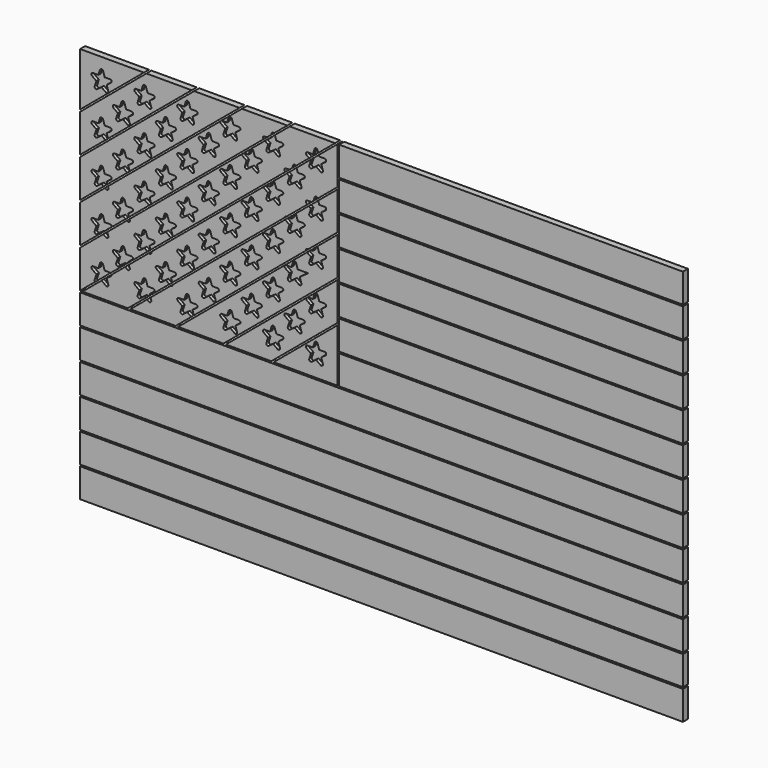
from build123d import *

# Parameters (mm, degrees)
F0_W     = 1219.2
F0_H     = 58.7375
F3_DEPTH = 12.7
F0_W_2   = 695.325
F4_START = 6.35
F4_DEPTH = 8.89
F5_R     = 3.175
F5_2_R   = 3.175
F5_3_R   = 3.175
F5_4_R   = 3.175
F5_5_R   = 3.175
F5_6_R   = 3.175
F5_7_R   = 3.175
F5_8_R   = 3.175
F5_9_R   = 3.175
F5_10_R  = 3.175
F5_11_R  = 3.175
F5_12_R  = 3.175
F5_13_R  = 3.175
F5_14_R  = 3.175
F5_15_R  = 3.175
F5_16_R  = 3.175
F5_17_R  = 3.175
F5_18_R  = 3.175
F5_19_R  = 3.175
F5_20_R  = 3.175
F5_21_R  = 3.175
F5_22_R  = 3.175
F5_23_R  = 3.175
F5_24_R  = 3.175
F5_25_R  = 3.175
F5_26_R  = 3.175
F5_27_R  = 3.175
F5_28_R  = 3.175
F5_29_R  = 3.175
F5_30_R  = 3.175
F5_31_R  = 3.175
F5_32_R  = 3.175
F5_33_R  = 3.175
F5_34_R  = 3.175
F5_35_R  = 3.175
F5_36_R  = 3.175
F5_37_R  = 3.175
F5_38_R  = 3.175
F5_39_R  = 3.175
F5_40_R  = 3.175
F5_41_R  = 3.175
F5_42_R  = 3.175
F5_43_R  = 3.175
F5_44_R  = 3.175
F5_45_R  = 3.175
F5_46_R  = 3.175
F5_47_R  = 3.175
F5_48_R  = 3.175
F5_49_R  = 3.175
F5_50_R  = 3.175


# Not quite as in the source:
# - a feature names something its author has since deleted; it is built from what else it names


with BuildPart() as f3:
    # F0 (on Front) → F3 (new body)
    with BuildSketch(Plane.XZ):
        with Locations((609.6, 277.01875)):
            Rectangle(F0_W, F0_H)
    extrude(amount=F3_DEPTH)


with BuildPart() as f3b:
    # F0 (on Front) → F3, piece 2 (new body)
    with BuildSketch(Plane.XZ):
        with Locations((609.6, 215.10625)):
            Rectangle(F0_W, F0_H)
    extrude(amount=F3_DEPTH)


with BuildPart() as f3c:
    # F0 (on Front) → F3, piece 3 (new body)
    with BuildSketch(Plane.XZ):
        with Locations((609.6, 153.19375)):
            Rectangle(F0_W, F0_H)
    extrude(amount=F3_DEPTH)


with BuildPart() as f3d:
    # F0 (on Front) → F3, piece 4 (new body)
    with BuildSketch(Plane.XZ):
        with Locations((609.6, 91.28125)):
            Rectangle(F0_W, F0_H)
    extrude(amount=F3_DEPTH)


with BuildPart() as f3e:
    # F0 (on Front) → F3, piece 5 (new body)
    with BuildSketch(Plane.XZ):
        with Locations((609.6, 29.36875)):
            Rectangle(F0_W, F0_H)
    extrude(amount=F3_DEPTH)


with BuildPart() as f3f:
    # F0 (on Front) → F3, piece 6 (new body)
    with BuildSketch(Plane.XZ):
        with Locations((609.6, 338.93125)):
            Rectangle(F0_W, F0_H)
    extrude(amount=F3_DEPTH)


with BuildPart() as f3g:
    # F0 (on Front) → F3, piece 7 (new body)
    with BuildSketch(Plane.XZ):
        with Locations((871.5375, 400.84375)):
            Rectangle(F0_W_2, F0_H)
    extrude(amount=F3_DEPTH)


with BuildPart() as f3h:
    # F0 (on Front) → F3, piece 8 (new body)
    with BuildSketch(Plane.XZ):
        with Locations((871.5375, 462.75625)):
            Rectangle(F0_W_2, F0_H)
    extrude(amount=F3_DEPTH)


with BuildPart() as f3i:
    # F0 (on Front) → F3, piece 9 (new body)
    with BuildSketch(Plane.XZ):
        with Locations((871.5375, 524.66875)):
            Rectangle(F0_W_2, F0_H)
    extrude(amount=F3_DEPTH)


with BuildPart() as f3j:
    # F0 (on Front) → F3, piece 10 (new body)
    with BuildSketch(Plane.XZ):
        with Locations((871.5375, 586.58125)):
            Rectangle(F0_W_2, F0_H)
    extrude(amount=F3_DEPTH)


with BuildPart() as f3k:
    # F0 (on Front) → F3, piece 11 (new body)
    with BuildSketch(Plane.XZ):
        with Locations((871.5375, 648.49375)):
            Rectangle(F0_W_2, F0_H)
    extrude(amount=F3_DEPTH)


with BuildPart() as f3l:
    # F0 (on Front) → F3, piece 12 (new body)
    with BuildSketch(Plane.XZ):
        with Locations((871.5375, 710.40625)):
            Rectangle(F0_W_2, F0_H)
    extrude(amount=F3_DEPTH)


with BuildPart() as f3m:
    # F0 (on Front) → F3, piece 13 (new body)
    with BuildSketch(Plane.XZ):
        with Locations((871.5375, 772.31875)):
            Rectangle(F0_W_2, F0_H)
    extrude(amount=F3_DEPTH)


with BuildPart() as f3n:
    # F0 (on Front) → F3, piece 14 (new body)
    with BuildSketch(Plane.XZ):
        Polygon((520.7, 371.475), (520.7, 479.188347446), (391.5720757397, 371.475), align=None)
    extrude(amount=F3_DEPTH)


with BuildPart() as f3o:
    # F0 (on Front) → F3, piece 15 (new body)
    with BuildSketch(Plane.XZ):
        Polygon((386.6154671861, 371.475), (520.7, 483.3229519659), (520.7, 559.8131355845), (294.9182089432, 371.475), align=None)
    extrude(amount=F3_DEPTH)


with BuildPart() as f3p:
    # F0 (on Front) → F3, piece 16 (new body)
    with BuildSketch(Plane.XZ):
        Polygon((520.7, 563.9477401044), (520.7, 640.437923723), (198.2643421467, 371.475), (289.9616003895, 371.475), align=None)
    extrude(amount=F3_DEPTH)


with BuildPart() as f3q:
    # F0 (on Front) → F3, piece 17 (new body)
    with BuildSketch(Plane.XZ):
        Polygon((520.7, 644.5725282429), (520.7, 721.0627118615), (101.6104753502, 371.475), (193.307733593, 371.475), align=None)
    extrude(amount=F3_DEPTH)


with BuildPart() as f3r:
    # F0 (on Front) → F3, piece 18 (new body)
    with BuildSketch(Plane.XZ):
        Polygon((520.7, 725.1973163814), (520.7, 801.6875), (4.9566085537, 371.475), (96.6538667965, 371.475), align=None)
    extrude(amount=F3_DEPTH)


with BuildPart() as f3s:
    # F0 (on Front) → F3, piece 19 (new body)
    with BuildSketch(Plane.XZ):
        Polygon((0, 371.475), (515.7433914463, 801.6875), (424.0461332035, 801.6875), (0, 447.9651836186), align=None)
    extrude(amount=F3_DEPTH)


with BuildPart() as f3t:
    # F0 (on Front) → F3, piece 20 (new body)
    with BuildSketch(Plane.XZ):
        Polygon((0, 528.5899717571), (0, 452.0997881385), (419.0895246498, 801.6875), (327.392266407, 801.6875), align=None)
    extrude(amount=F3_DEPTH)


with BuildPart() as f3u:
    # F0 (on Front) → F3, piece 21 (new body)
    with BuildSketch(Plane.XZ):
        Polygon((0, 532.724576277), (322.4356578533, 801.6875), (230.7383996105, 801.6875), (0, 609.2147598956), align=None)
    extrude(amount=F3_DEPTH)


with BuildPart() as f3v:
    # F0 (on Front) → F3, piece 22 (new body)
    with BuildSketch(Plane.XZ):
        Polygon((0, 613.3493644155), (225.7817910568, 801.6875), (134.0845328139, 801.6875), (0, 689.8395480341), align=None)
    extrude(amount=F3_DEPTH)


with BuildPart() as f3w:
    # F0 (on Front) → F3, piece 23 (new body)
    with BuildSketch(Plane.XZ):
        Polygon((0, 693.974152554), (129.1279242603, 801.6875), (0, 801.6875), align=None)
    extrude(amount=F3_DEPTH)


with BuildPart() as f4:
    # F2 (on Front) → F4 (new body)
    with BuildSketch(Plane.XZ.offset(F4_START)):
        Polygon((69.9856764157, 606.4772193857), (86.78164, 618.6802012285), (103.5776035843, 606.4772193857), (97.1621163689, 626.2220587715), (113.9580799531, 638.4250406143), (93.1971272154, 638.4250406143), (86.78164, 658.16988), (80.3661527846, 638.4250406143), (59.6052000469, 638.4250406143), (76.4011636311, 626.2220587715), align=None)
    extrude(amount=F4_DEPTH)

    # F5#35
    f5_35_edges = [f4.edges().sort_by_distance(p)[0] for p in [
        (59.6052, -10.795, 638.425041),
        (103.577604, -10.795, 606.477219),
        (86.78164, -10.795, 658.16988),
        (113.95808, -10.795, 638.425041),
        (69.985676, -10.795, 606.477219),
    ]]
    fillet(f5_35_edges, radius=F5_35_R)


with BuildPart() as f4b:
    # F2 (on Front) → F4, piece 2 (new body)
    with BuildSketch(Plane.XZ.offset(F4_START)):
        Polygon((26.5948564157, 735.5371593857), (43.39082, 747.7401412285), (60.1867835842, 735.5371593857), (53.7712963689, 755.2819987715), (70.5672599531, 767.4849806143), (49.8063072154, 767.4849806143), (43.39082, 787.22982), (36.9753327846, 767.4849806143), (16.2143800469, 767.4849806143), (33.0103436311, 755.2819987715), align=None)
    extrude(amount=F4_DEPTH)

    # F5#33
    f5_33_edges = [f4b.edges().sort_by_distance(p)[0] for p in [
        (70.56726, -10.795, 767.484981),
        (26.594856, -10.795, 735.537159),
        (60.186784, -10.795, 735.537159),
        (16.21438, -10.795, 767.484981),
        (43.39082, -10.795, 787.22982),
    ]]
    fillet(f5_33_edges, radius=F5_33_R)


with BuildPart() as f4c:
    # F2 (on Front) → F4, piece 3 (new body)
    with BuildSketch(Plane.XZ.offset(F4_START)):
        Polygon((113.3764964157, 735.5371593857), (130.17246, 747.7401412285), (146.9684235843, 735.5371593857), (140.5529363689, 755.2819987715), (157.3488999531, 767.4849806142), (136.5879472154, 767.4849806143), (130.17246, 787.22982), (123.7569727846, 767.4849806143), (102.9960200469, 767.4849806143), (119.7919836311, 755.2819987715), align=None)
    extrude(amount=F4_DEPTH)

    # F5#29
    f5_29_edges = [f4c.edges().sort_by_distance(p)[0] for p in [
        (157.3489, -10.795, 767.484981),
        (146.968424, -10.795, 735.537159),
        (113.376496, -10.795, 735.537159),
        (130.17246, -10.795, 787.22982),
        (102.99602, -10.795, 767.484981),
    ]]
    fillet(f5_29_edges, radius=F5_29_R)


with BuildPart() as f4d:
    # F2 (on Front) → F4, piece 4 (new body)
    with BuildSketch(Plane.XZ.offset(F4_START)):
        Polygon((200.1581364157, 735.5371593857), (216.9541, 747.7401412285), (233.7500635843, 735.5371593857), (227.3345763689, 755.2819987715), (244.1305399531, 767.4849806143), (223.3695872154, 767.4849806143), (216.9541, 787.22982), (210.5386127846, 767.4849806143), (189.7776600469, 767.4849806143), (206.5736236311, 755.2819987715), align=None)
    extrude(amount=F4_DEPTH)

    # F5#27
    f5_27_edges = [f4d.edges().sort_by_distance(p)[0] for p in [
        (244.13054, -10.795, 767.484981),
        (216.9541, -10.795, 787.22982),
        (233.750064, -10.795, 735.537159),
        (200.158136, -10.795, 735.537159),
        (189.77766, -10.795, 767.484981),
    ]]
    fillet(f5_27_edges, radius=F5_27_R)


with BuildPart() as f4e:
    # F2 (on Front) → F4, piece 5 (new body)
    with BuildSketch(Plane.XZ.offset(F4_START)):
        Polygon((286.9397764157, 735.5371593857), (303.73574, 747.7401412285), (320.5317035842, 735.5371593857), (314.1162163689, 755.2819987715), (330.9121799531, 767.4849806143), (310.1512272154, 767.4849806143), (303.73574, 787.22982), (297.3202527846, 767.4849806143), (276.5593000469, 767.4849806143), (293.3552636311, 755.2819987715), align=None)
    extrude(amount=F4_DEPTH)

    # F5#5
    f5_5_edges = [f4e.edges().sort_by_distance(p)[0] for p in [
        (330.91218, -10.795, 767.484981),
        (320.531704, -10.795, 735.537159),
        (286.939776, -10.795, 735.537159),
        (303.73574, -10.795, 787.22982),
        (276.5593, -10.795, 767.484981),
    ]]
    fillet(f5_5_edges, radius=F5_5_R)


with BuildPart() as f4f:
    # F2 (on Front) → F4, piece 6 (new body)
    with BuildSketch(Plane.XZ.offset(F4_START)):
        Polygon((373.7214164157, 735.5371593857), (390.51738, 747.7401412285), (407.3133435843, 735.5371593857), (400.8978563689, 755.2819987715), (417.6938199531, 767.4849806143), (396.9328672154, 767.4849806143), (390.51738, 787.22982), (384.1018927846, 767.4849806142), (363.3409400469, 767.4849806143), (380.1369036311, 755.2819987715), align=None)
    extrude(amount=F4_DEPTH)

    # F5#2
    f5_2_edges = [f4f.edges().sort_by_distance(p)[0] for p in [
        (390.51738, -10.795, 787.22982),
        (407.313344, -10.795, 735.537159),
        (363.34094, -10.795, 767.484981),
        (373.721416, -10.795, 735.537159),
        (417.69382, -10.795, 767.484981),
    ]]
    fillet(f5_2_edges, radius=F5_2_R)


with BuildPart() as f4g:
    # F2 (on Front) → F4, piece 7 (new body)
    with BuildSketch(Plane.XZ.offset(F4_START)):
        Polygon((460.5030564157, 735.5371593857), (477.29902, 747.7401412285), (494.0949835843, 735.5371593857), (487.6794963689, 755.2819987715), (504.4754599531, 767.4849806143), (483.7145072154, 767.4849806143), (477.29902, 787.22982), (470.8835327846, 767.4849806143), (450.1225800469, 767.4849806143), (466.9185436311, 755.2819987715), align=None)
    extrude(amount=F4_DEPTH)

    # F5
    f5_edges = [f4g.edges().sort_by_distance(p)[0] for p in [
        (477.29902, -10.795, 787.22982),
        (504.47546, -10.795, 767.484981),
        (494.094984, -10.795, 735.537159),
        (460.503056, -10.795, 735.537159),
        (450.12258, -10.795, 767.484981),
    ]]
    fillet(f5_edges, radius=F5_R)


with BuildPart() as f4h:
    # F2 (on Front) → F4, piece 8 (new body)
    with BuildSketch(Plane.XZ.offset(F4_START)):
        Polygon((460.5030564157, 649.4971993857), (477.29902, 661.7001812285), (494.0949835843, 649.4971993857), (487.6794963689, 669.2420387715), (504.4754599531, 681.4450206143), (483.7145072154, 681.4450206143), (477.29902, 701.18986), (470.8835327846, 681.4450206143), (450.1225800469, 681.4450206143), (466.9185436311, 669.2420387715), align=None)
    extrude(amount=F4_DEPTH)

    # F5#3
    f5_3_edges = [f4h.edges().sort_by_distance(p)[0] for p in [
        (504.47546, -10.795, 681.445021),
        (477.29902, -10.795, 701.18986),
        (450.12258, -10.795, 681.445021),
        (460.503056, -10.795, 649.497199),
        (494.094984, -10.795, 649.497199),
    ]]
    fillet(f5_3_edges, radius=F5_3_R)


with BuildPart() as f4i:
    # F2 (on Front) → F4, piece 9 (new body)
    with BuildSketch(Plane.XZ.offset(F4_START)):
        Polygon((417.1122364157, 692.5171793858), (433.9082, 704.7201612285), (450.7041635842, 692.5171793857), (444.2886763689, 712.2620187715), (461.0846399531, 724.4650006143), (440.3236872154, 724.4650006143), (433.9082, 744.20984), (427.4927127846, 724.4650006143), (406.7317600469, 724.4650006143), (423.5277236311, 712.2620187715), align=None)
    extrude(amount=F4_DEPTH)

    # F5#4
    f5_4_edges = [f4i.edges().sort_by_distance(p)[0] for p in [
        (433.9082, -10.795, 744.20984),
        (406.73176, -10.795, 724.465001),
        (450.704164, -10.795, 692.517179),
        (461.08464, -10.795, 724.465001),
        (417.112236, -10.795, 692.517179),
    ]]
    fillet(f5_4_edges, radius=F5_4_R)


with BuildPart() as f4j:
    # F2 (on Front) → F4, piece 10 (new body)
    with BuildSketch(Plane.XZ.offset(F4_START)):
        Polygon((113.3764964157, 649.4971993857), (130.17246, 661.7001812285), (146.9684235843, 649.4971993857), (140.5529363689, 669.2420387715), (157.3488999531, 681.4450206143), (136.5879472154, 681.4450206143), (130.17246, 701.18986), (123.7569727846, 681.4450206143), (102.9960200469, 681.4450206143), (119.7919836311, 669.2420387715), align=None)
    extrude(amount=F4_DEPTH)

    # F5#31
    f5_31_edges = [f4j.edges().sort_by_distance(p)[0] for p in [
        (157.3489, -10.795, 681.445021),
        (130.17246, -10.795, 701.18986),
        (146.968424, -10.795, 649.497199),
        (102.99602, -10.795, 681.445021),
        (113.376496, -10.795, 649.497199),
    ]]
    fillet(f5_31_edges, radius=F5_31_R)


with BuildPart() as f4k:
    # F2 (on Front) → F4, piece 11 (new body)
    with BuildSketch(Plane.XZ.offset(F4_START)):
        Polygon((156.7673164157, 520.4372593857), (173.56328, 532.6402412285), (190.3592435843, 520.4372593857), (183.9437563689, 540.1820987715), (200.7397199531, 552.3850806143), (179.9787672154, 552.3850806143), (173.56328, 572.12992), (167.1477927846, 552.3850806143), (146.3868400469, 552.3850806143), (163.1828036311, 540.1820987715), align=None)
    extrude(amount=F4_DEPTH)

    # F5#37
    f5_37_edges = [f4k.edges().sort_by_distance(p)[0] for p in [
        (173.56328, -10.795, 572.12992),
        (146.38684, -10.795, 552.385081),
        (156.767316, -10.795, 520.437259),
        (190.359244, -10.795, 520.437259),
        (200.73972, -10.795, 552.385081),
    ]]
    fillet(f5_37_edges, radius=F5_37_R)


with BuildPart() as f4l:
    # F2 (on Front) → F4, piece 12 (new body)
    with BuildSketch(Plane.XZ.offset(F4_START)):
        Polygon((26.5948564157, 649.4971993857), (43.39082, 661.7001812285), (60.1867835843, 649.4971993857), (53.7712963689, 669.2420387715), (70.5672599531, 681.4450206143), (49.8063072154, 681.4450206143), (43.39082, 701.18986), (36.9753327846, 681.4450206143), (16.2143800469, 681.4450206143), (33.0103436311, 669.2420387715), align=None)
    extrude(amount=F4_DEPTH)

    # F5#34
    f5_34_edges = [f4l.edges().sort_by_distance(p)[0] for p in [
        (16.21438, -10.795, 681.445021),
        (43.39082, -10.795, 701.18986),
        (60.186784, -10.795, 649.497199),
        (26.594856, -10.795, 649.497199),
        (70.56726, -10.795, 681.445021),
    ]]
    fillet(f5_34_edges, radius=F5_34_R)


with BuildPart() as f4m:
    # F2 (on Front) → F4, piece 13 (new body)
    with BuildSketch(Plane.XZ.offset(F4_START)):
        Polygon((200.1581364158, 477.4172793857), (216.9541, 489.6202612285), (233.7500635843, 477.4172793857), (227.3345763689, 497.1621187715), (244.1305399531, 509.3651006143), (223.3695872154, 509.3651006143), (216.9541, 529.10994), (210.5386127846, 509.3651006143), (189.7776600469, 509.3651006143), (206.5736236311, 497.1621187715), align=None)
    extrude(amount=F4_DEPTH)

    # F5#42
    f5_42_edges = [f4m.edges().sort_by_distance(p)[0] for p in [
        (189.77766, -10.795, 509.365101),
        (216.9541, -10.795, 529.10994),
        (233.750064, -10.795, 477.417279),
        (200.158136, -10.795, 477.417279),
        (244.13054, -10.795, 509.365101),
    ]]
    fillet(f5_42_edges, radius=F5_42_R)


with BuildPart() as f4n:
    # F2 (on Front) → F4, piece 14 (new body)
    with BuildSketch(Plane.XZ.offset(F4_START)):
        Polygon((460.5030564157, 563.4572393857), (477.29902, 575.6602212285), (494.0949835843, 563.4572393857), (487.6794963689, 583.2020787715), (504.4754599531, 595.4050606143), (483.7145072154, 595.4050606143), (477.29902, 615.1499), (470.8835327846, 595.4050606143), (450.1225800469, 595.4050606143), (466.9185436311, 583.2020787715), align=None)
    extrude(amount=F4_DEPTH)

    # F5#14
    f5_14_edges = [f4n.edges().sort_by_distance(p)[0] for p in [
        (477.29902, -10.795, 615.1499),
        (504.47546, -10.795, 595.405061),
        (450.12258, -10.795, 595.405061),
        (494.094984, -10.795, 563.457239),
        (460.503056, -10.795, 563.457239),
    ]]
    fillet(f5_14_edges, radius=F5_14_R)


with BuildPart() as f4o:
    # F2 (on Front) → F4, piece 15 (new body)
    with BuildSketch(Plane.XZ.offset(F4_START)):
        Polygon((417.1122364157, 434.3972993857), (433.9082, 446.6002812285), (450.7041635843, 434.3972993857), (444.2886763689, 454.1421387715), (461.0846399531, 466.3451206143), (440.3236872154, 466.3451206143), (433.9082, 486.08996), (427.4927127846, 466.3451206143), (406.7317600469, 466.3451206143), (423.5277236311, 454.1421387715), align=None)
    extrude(amount=F4_DEPTH)

    # F5#12
    f5_12_edges = [f4o.edges().sort_by_distance(p)[0] for p in [
        (433.9082, -10.795, 486.08996),
        (461.08464, -10.795, 466.345121),
        (450.704164, -10.795, 434.397299),
        (406.73176, -10.795, 466.345121),
        (417.112236, -10.795, 434.397299),
    ]]
    fillet(f5_12_edges, radius=F5_12_R)


with BuildPart() as f4p:
    # F2 (on Front) → F4, piece 16 (new body)
    with BuildSketch(Plane.XZ.offset(F4_START)):
        Polygon((113.3764964157, 391.3773193857), (130.17246, 403.5803012285), (146.9684235843, 391.3773193857), (140.5529363689, 411.1221587715), (157.3488999531, 423.3251406143), (136.5879472154, 423.3251406143), (130.17246, 443.06998), (123.7569727846, 423.3251406143), (102.9960200469, 423.3251406143), (119.7919836311, 411.1221587715), align=None)
    extrude(amount=F4_DEPTH)

    # F5#44
    f5_44_edges = [f4p.edges().sort_by_distance(p)[0] for p in [
        (146.968424, -10.795, 391.377319),
        (113.376496, -10.795, 391.377319),
        (157.3489, -10.795, 423.325141),
        (130.17246, -10.795, 443.06998),
        (102.99602, -10.795, 423.325141),
    ]]
    fillet(f5_44_edges, radius=F5_44_R)


with BuildPart() as f4q:
    # F2 (on Front) → F4, piece 17 (new body)
    with BuildSketch(Plane.XZ.offset(F4_START)):
        Polygon((373.7214164157, 649.4971993857), (390.51738, 661.7001812285), (407.3133435843, 649.4971993857), (400.8978563689, 669.2420387715), (417.6938199531, 681.4450206143), (396.9328672154, 681.4450206143), (390.51738, 701.18986), (384.1018927846, 681.4450206143), (363.3409400469, 681.4450206143), (380.1369036311, 669.2420387715), align=None)
    extrude(amount=F4_DEPTH)

    # F5#8
    f5_8_edges = [f4q.edges().sort_by_distance(p)[0] for p in [
        (363.34094, -10.795, 681.445021),
        (417.69382, -10.795, 681.445021),
        (390.51738, -10.795, 701.18986),
        (373.721416, -10.795, 649.497199),
        (407.313344, -10.795, 649.497199),
    ]]
    fillet(f5_8_edges, radius=F5_8_R)


with BuildPart() as f4r:
    # F2 (on Front) → F4, piece 18 (new body)
    with BuildSketch(Plane.XZ.offset(F4_START)):
        Polygon((200.1581364157, 649.4971993857), (216.9541, 661.7001812285), (233.7500635843, 649.4971993857), (227.3345763689, 669.2420387715), (244.1305399531, 681.4450206143), (223.3695872154, 681.4450206143), (216.9541, 701.18986), (210.5386127846, 681.4450206143), (189.7776600469, 681.4450206143), (206.5736236311, 669.2420387715), align=None)
    extrude(amount=F4_DEPTH)

    # F5#26
    f5_26_edges = [f4r.edges().sort_by_distance(p)[0] for p in [
        (244.13054, -10.795, 681.445021),
        (216.9541, -10.795, 701.18986),
        (189.77766, -10.795, 681.445021),
        (200.158136, -10.795, 649.497199),
        (233.750064, -10.795, 649.497199),
    ]]
    fillet(f5_26_edges, radius=F5_26_R)


with BuildPart() as f4s:
    # F2 (on Front) → F4, piece 19 (new body)
    with BuildSketch(Plane.XZ.offset(F4_START)):
        Polygon((286.9397764157, 649.4971993857), (303.73574, 661.7001812285), (320.5317035843, 649.4971993857), (314.1162163689, 669.2420387715), (330.9121799531, 681.4450206143), (310.1512272154, 681.4450206143), (303.73574, 701.18986), (297.3202527846, 681.4450206143), (276.5593000469, 681.4450206143), (293.3552636311, 669.2420387715), align=None)
    extrude(amount=F4_DEPTH)

    # F5#19
    f5_19_edges = [f4s.edges().sort_by_distance(p)[0] for p in [
        (320.531704, -10.795, 649.497199),
        (330.91218, -10.795, 681.445021),
        (286.939776, -10.795, 649.497199),
        (276.5593, -10.795, 681.445021),
        (303.73574, -10.795, 701.18986),
    ]]
    fillet(f5_19_edges, radius=F5_19_R)


with BuildPart() as f4t:
    # F2 (on Front) → F4, piece 20 (new body)
    with BuildSketch(Plane.XZ.offset(F4_START)):
        Polygon((243.5489564157, 692.5171793857), (260.34492, 704.7201612285), (277.1408835843, 692.5171793857), (270.7253963689, 712.2620187715), (287.5213599531, 724.4650006143), (266.7604072154, 724.4650006143), (260.34492, 744.20984), (253.9294327846, 724.4650006143), (233.1684800469, 724.4650006143), (249.9644436311, 712.2620187715), align=None)
    extrude(amount=F4_DEPTH)

    # F5#23
    f5_23_edges = [f4t.edges().sort_by_distance(p)[0] for p in [
        (287.52136, -10.795, 724.465001),
        (277.140884, -10.795, 692.517179),
        (260.34492, -10.795, 744.20984),
        (233.16848, -10.795, 724.465001),
        (243.548956, -10.795, 692.517179),
    ]]
    fillet(f5_23_edges, radius=F5_23_R)


with BuildPart() as f4u:
    # F2 (on Front) → F4, piece 21 (new body)
    with BuildSketch(Plane.XZ.offset(F4_START)):
        Polygon((330.3305964157, 692.5171793857), (347.12656, 704.7201612285), (363.9225235842, 692.5171793857), (357.5070363689, 712.2620187715), (374.3029999531, 724.4650006143), (353.5420472154, 724.4650006143), (347.12656, 744.20984), (340.7110727846, 724.4650006143), (319.9501200469, 724.4650006143), (336.7460836311, 712.2620187715), align=None)
    extrude(amount=F4_DEPTH)

    # F5#6
    f5_6_edges = [f4u.edges().sort_by_distance(p)[0] for p in [
        (347.12656, -10.795, 744.20984),
        (319.95012, -10.795, 724.465001),
        (374.303, -10.795, 724.465001),
        (330.330596, -10.795, 692.517179),
        (363.922524, -10.795, 692.517179),
    ]]
    fillet(f5_6_edges, radius=F5_6_R)


with BuildPart() as f4v:
    # F2 (on Front) → F4, piece 22 (new body)
    with BuildSketch(Plane.XZ.offset(F4_START)):
        Polygon((156.7673164157, 692.5171793857), (173.56328, 704.7201612285), (190.3592435842, 692.5171793857), (183.9437563689, 712.2620187715), (200.7397199531, 724.4650006143), (179.9787672154, 724.4650006143), (173.56328, 744.20984), (167.1477927846, 724.4650006143), (146.3868400469, 724.4650006143), (163.1828036311, 712.2620187715), align=None)
    extrude(amount=F4_DEPTH)

    # F5#28
    f5_28_edges = [f4v.edges().sort_by_distance(p)[0] for p in [
        (200.73972, -10.795, 724.465001),
        (173.56328, -10.795, 744.20984),
        (146.38684, -10.795, 724.465001),
        (190.359244, -10.795, 692.517179),
        (156.767316, -10.795, 692.517179),
    ]]
    fillet(f5_28_edges, radius=F5_28_R)


with BuildPart() as f4w:
    # F2 (on Front) → F4, piece 23 (new body)
    with BuildSketch(Plane.XZ.offset(F4_START)):
        Polygon((373.7214164158, 563.4572393857), (390.51738, 575.6602212285), (407.3133435843, 563.4572393857), (400.8978563689, 583.2020787715), (417.6938199531, 595.4050606143), (396.9328672154, 595.4050606143), (390.51738, 615.1499), (384.1018927846, 595.4050606143), (363.3409400469, 595.4050606143), (380.1369036311, 583.2020787715), align=None)
    extrude(amount=F4_DEPTH)

    # F5#9
    f5_9_edges = [f4w.edges().sort_by_distance(p)[0] for p in [
        (390.51738, -10.795, 615.1499),
        (407.313344, -10.795, 563.457239),
        (417.69382, -10.795, 595.405061),
        (373.721416, -10.795, 563.457239),
        (363.34094, -10.795, 595.405061),
    ]]
    fillet(f5_9_edges, radius=F5_9_R)


with BuildPart() as f4x:
    # F2 (on Front) → F4, piece 24 (new body)
    with BuildSketch(Plane.XZ.offset(F4_START)):
        Polygon((200.1581364157, 563.4572393858), (216.9541, 575.6602212285), (233.7500635843, 563.4572393857), (227.3345763689, 583.2020787715), (244.1305399531, 595.4050606143), (223.3695872154, 595.4050606143), (216.9541, 615.1499), (210.5386127846, 595.4050606143), (189.7776600469, 595.4050606143), (206.5736236311, 583.2020787715), align=None)
    extrude(amount=F4_DEPTH)

    # F5#22
    f5_22_edges = [f4x.edges().sort_by_distance(p)[0] for p in [
        (216.9541, -10.795, 615.1499),
        (244.13054, -10.795, 595.405061),
        (189.77766, -10.795, 595.405061),
        (200.158136, -10.795, 563.457239),
        (233.750064, -10.795, 563.457239),
    ]]
    fillet(f5_22_edges, radius=F5_22_R)


with BuildPart() as f4y:
    # F2 (on Front) → F4, piece 25 (new body)
    with BuildSketch(Plane.XZ.offset(F4_START)):
        Polygon((69.9856764157, 692.5171793857), (86.78164, 704.7201612285), (103.5776035843, 692.5171793857), (97.1621163689, 712.2620187715), (113.9580799531, 724.4650006143), (93.1971272154, 724.4650006143), (86.78164, 744.20984), (80.3661527846, 724.4650006143), (59.6052000469, 724.4650006143), (76.4011636311, 712.2620187715), align=None)
    extrude(amount=F4_DEPTH)

    # F5#30
    f5_30_edges = [f4y.edges().sort_by_distance(p)[0] for p in [
        (113.95808, -10.795, 724.465001),
        (86.78164, -10.795, 744.20984),
        (103.577604, -10.795, 692.517179),
        (69.985676, -10.795, 692.517179),
        (59.6052, -10.795, 724.465001),
    ]]
    fillet(f5_30_edges, radius=F5_30_R)


with BuildPart() as f4z:
    # F2 (on Front) → F4, piece 26 (new body)
    with BuildSketch(Plane.XZ.offset(F4_START)):
        Polygon((460.5030564157, 477.4172793857), (477.29902, 489.6202612285), (494.0949835843, 477.4172793857), (487.6794963689, 497.1621187715), (504.4754599531, 509.3651006143), (483.7145072154, 509.3651006143), (477.29902, 529.10994), (470.8835327846, 509.3651006143), (450.1225800469, 509.3651006143), (466.9185436311, 497.1621187715), align=None)
    extrude(amount=F4_DEPTH)

    # F5#13
    f5_13_edges = [f4z.edges().sort_by_distance(p)[0] for p in [
        (450.12258, -10.795, 509.365101),
        (477.29902, -10.795, 529.10994),
        (494.094984, -10.795, 477.417279),
        (460.503056, -10.795, 477.417279),
        (504.47546, -10.795, 509.365101),
    ]]
    fillet(f5_13_edges, radius=F5_13_R)


with BuildPart() as f4ba:
    # F2 (on Front) → F4, piece 27 (new body)
    with BuildSketch(Plane.XZ.offset(F4_START)):
        Polygon((417.1122364158, 520.4372593857), (433.9082, 532.6402412285), (450.7041635843, 520.4372593857), (444.2886763689, 540.1820987715), (461.0846399531, 552.3850806143), (440.3236872154, 552.3850806143), (433.9082, 572.12992), (427.4927127846, 552.3850806143), (406.7317600469, 552.3850806143), (423.5277236311, 540.1820987715), align=None)
    extrude(amount=F4_DEPTH)

    # F5#11
    f5_11_edges = [f4ba.edges().sort_by_distance(p)[0] for p in [
        (433.9082, -10.795, 572.12992),
        (450.704164, -10.795, 520.437259),
        (417.112236, -10.795, 520.437259),
        (406.73176, -10.795, 552.385081),
    ]]
    fillet(f5_11_edges, radius=F5_11_R)


with BuildPart() as f4bb:
    # F2 (on Front) → F4, piece 28 (new body)
    with BuildSketch(Plane.XZ.offset(F4_START)):
        Polygon((113.3764964158, 477.4172793857), (130.17246, 489.6202612285), (146.9684235843, 477.4172793857), (140.5529363689, 497.1621187715), (157.3488999531, 509.3651006143), (136.5879472154, 509.3651006143), (130.17246, 529.10994), (123.7569727846, 509.3651006143), (102.9960200469, 509.3651006143), (119.7919836311, 497.1621187715), align=None)
    extrude(amount=F4_DEPTH)

    # F5#41
    f5_41_edges = [f4bb.edges().sort_by_distance(p)[0] for p in [
        (102.99602, -10.795, 509.365101),
        (146.968424, -10.795, 477.417279),
        (157.3489, -10.795, 509.365101),
        (113.376496, -10.795, 477.417279),
        (130.17246, -10.795, 529.10994),
    ]]
    fillet(f5_41_edges, radius=F5_41_R)


with BuildPart() as f4bc:
    # F2 (on Front) → F4, piece 29 (new body)
    with BuildSketch(Plane.XZ.offset(F4_START)):
        Polygon((26.5948564157, 391.3773193857), (43.39082, 403.5803012285), (60.1867835843, 391.3773193857), (53.7712963689, 411.1221587715), (70.5672599531, 423.3251406143), (49.8063072154, 423.3251406143), (43.39082, 443.06998), (36.9753327846, 423.3251406143), (16.2143800469, 423.3251406143), (33.0103436311, 411.1221587715), align=None)
    extrude(amount=F4_DEPTH)

    # F5#45
    f5_45_edges = [f4bc.edges().sort_by_distance(p)[0] for p in [
        (60.186784, -10.795, 391.377319),
        (26.594856, -10.795, 391.377319),
        (16.21438, -10.795, 423.325141),
        (70.56726, -10.795, 423.325141),
        (43.39082, -10.795, 443.06998),
    ]]
    fillet(f5_45_edges, radius=F5_45_R)


with BuildPart() as f4bd:
    # F2 (on Front) → F4, piece 30 (new body)
    with BuildSketch(Plane.XZ.offset(F4_START)):
        Polygon((330.3305964157, 520.4372593857), (347.12656, 532.6402412285), (363.9225235842, 520.4372593857), (357.5070363689, 540.1820987715), (374.3029999531, 552.3850806143), (353.5420472154, 552.3850806143), (347.12656, 572.12992), (340.7110727846, 552.3850806143), (319.9501200469, 552.3850806143), (336.7460836311, 540.1820987715), align=None)
    extrude(amount=F4_DEPTH)

    # F5#18
    f5_18_edges = [f4bd.edges().sort_by_distance(p)[0] for p in [
        (347.12656, -10.795, 572.12992),
        (363.922524, -10.795, 520.437259),
        (374.303, -10.795, 552.385081),
        (330.330596, -10.795, 520.437259),
        (319.95012, -10.795, 552.385081),
    ]]
    fillet(f5_18_edges, radius=F5_18_R)


with BuildPart() as f4be:
    # F2 (on Front) → F4, piece 31 (new body)
    with BuildSketch(Plane.XZ.offset(F4_START)):
        Polygon((373.7214164157, 477.4172793858), (390.51738, 489.6202612285), (407.3133435843, 477.4172793857), (400.8978563689, 497.1621187715), (417.6938199531, 509.3651006143), (396.9328672154, 509.3651006143), (390.51738, 529.10994), (384.1018927846, 509.3651006143), (363.3409400469, 509.3651006143), (380.1369036311, 497.1621187715), align=None)
    extrude(amount=F4_DEPTH)

    # F5#15
    f5_15_edges = [f4be.edges().sort_by_distance(p)[0] for p in [
        (390.51738, -10.795, 529.10994),
        (373.721416, -10.795, 477.417279),
        (407.313344, -10.795, 477.417279),
        (417.69382, -10.795, 509.365101),
        (363.34094, -10.795, 509.365101),
    ]]
    fillet(f5_15_edges, radius=F5_15_R)


with BuildPart() as f4bf:
    # F2 (on Front) → F4, piece 32 (new body)
    with BuildSketch(Plane.XZ.offset(F4_START)):
        Polygon((69.9856764157, 434.3972993857), (86.78164, 446.6002812285), (103.5776035843, 434.3972993857), (97.1621163689, 454.1421387715), (113.9580799531, 466.3451206143), (93.1971272154, 466.3451206143), (86.78164, 486.08996), (80.3661527846, 466.3451206143), (59.6052000469, 466.3451206143), (76.4011636311, 454.1421387715), align=None)
    extrude(amount=F4_DEPTH)

    # F5#46
    f5_46_edges = [f4bf.edges().sort_by_distance(p)[0] for p in [
        (103.577604, -10.795, 434.397299),
        (113.95808, -10.795, 466.345121),
        (59.6052, -10.795, 466.345121),
        (69.985676, -10.795, 434.397299),
        (86.78164, -10.795, 486.08996),
    ]]
    fillet(f5_46_edges, radius=F5_46_R)


with BuildPart() as f4bg:
    # F2 (on Front) → F4, piece 33 (new body)
    with BuildSketch(Plane.XZ.offset(F4_START)):
        Polygon((286.9397764157, 477.4172793857), (303.73574, 489.6202612285), (320.5317035843, 477.4172793857), (314.1162163689, 497.1621187715), (330.9121799531, 509.3651006143), (310.1512272154, 509.3651006143), (303.73574, 529.10994), (297.3202527846, 509.3651006143), (276.5593000469, 509.3651006143), (293.3552636311, 497.1621187715), align=None)
    extrude(amount=F4_DEPTH)

    # F5#24
    f5_24_edges = [f4bg.edges().sort_by_distance(p)[0] for p in [
        (330.91218, -10.795, 509.365101),
        (276.5593, -10.795, 509.365101),
        (303.73574, -10.795, 529.10994),
        (320.531704, -10.795, 477.417279),
        (286.939776, -10.795, 477.417279),
    ]]
    fillet(f5_24_edges, radius=F5_24_R)


with BuildPart() as f4bh:
    # F2 (on Front) → F4, piece 34 (new body)
    with BuildSketch(Plane.XZ.offset(F4_START)):
        Polygon((113.3764964157, 563.4572393858), (130.17246, 575.6602212285), (146.9684235843, 563.4572393857), (140.5529363689, 583.2020787715), (157.3488999531, 595.4050606143), (136.5879472154, 595.4050606143), (130.17246, 615.1499), (123.7569727846, 595.4050606143), (102.9960200469, 595.4050606143), (119.7919836311, 583.2020787715), align=None)
    extrude(amount=F4_DEPTH)

    # F5#36
    f5_36_edges = [f4bh.edges().sort_by_distance(p)[0] for p in [
        (130.17246, -10.795, 615.1499),
        (102.99602, -10.795, 595.405061),
        (113.376496, -10.795, 563.457239),
        (146.968424, -10.795, 563.457239),
        (157.3489, -10.795, 595.405061),
    ]]
    fillet(f5_36_edges, radius=F5_36_R)


with BuildPart() as f4bi:
    # F2 (on Front) → F4, piece 35 (new body)
    with BuildSketch(Plane.XZ.offset(F4_START)):
        Polygon((26.5948564157, 477.4172793857), (43.39082, 489.6202612285), (60.1867835843, 477.4172793857), (53.7712963689, 497.1621187715), (70.5672599531, 509.3651006143), (49.8063072154, 509.3651006143), (43.39082, 529.10994), (36.9753327846, 509.3651006143), (16.2143800469, 509.3651006143), (33.0103436311, 497.1621187715), align=None)
    extrude(amount=F4_DEPTH)

    # F5#40
    f5_40_edges = [f4bi.edges().sort_by_distance(p)[0] for p in [
        (16.21438, -10.795, 509.365101),
        (26.594856, -10.795, 477.417279),
        (43.39082, -10.795, 529.10994),
        (60.186784, -10.795, 477.417279),
        (70.56726, -10.795, 509.365101),
    ]]
    fillet(f5_40_edges, radius=F5_40_R)


with BuildPart() as f4bj:
    # F2 (on Front) → F4, piece 36 (new body)
    with BuildSketch(Plane.XZ.offset(F4_START)):
        Polygon((69.9856764157, 520.4372593857), (86.78164, 532.6402412285), (103.5776035843, 520.4372593857), (97.1621163689, 540.1820987715), (113.9580799531, 552.3850806143), (93.1971272154, 552.3850806143), (86.78164, 572.12992), (80.3661527846, 552.3850806143), (59.6052000469, 552.3850806143), (76.4011636311, 540.1820987715), align=None)
    extrude(amount=F4_DEPTH)

    # F5#39
    f5_39_edges = [f4bj.edges().sort_by_distance(p)[0] for p in [
        (59.6052, -10.795, 552.385081),
        (86.78164, -10.795, 572.12992),
        (69.985676, -10.795, 520.437259),
        (103.577604, -10.795, 520.437259),
        (113.95808, -10.795, 552.385081),
    ]]
    fillet(f5_39_edges, radius=F5_39_R)


with BuildPart() as f4bk:
    # F2 (on Front) → F4, piece 37 (new body)
    with BuildSketch(Plane.XZ.offset(F4_START)):
        Polygon((330.3305964157, 434.3972993858), (347.12656, 446.6002812285), (363.9225235843, 434.3972993857), (357.5070363689, 454.1421387715), (374.3029999531, 466.3451206143), (353.5420472154, 466.3451206143), (347.12656, 486.08996), (340.7110727846, 466.3451206143), (319.9501200469, 466.3451206143), (336.7460836311, 454.1421387715), align=None)
    extrude(amount=F4_DEPTH)

    # F5#17
    f5_17_edges = [f4bk.edges().sort_by_distance(p)[0] for p in [
        (347.12656, -10.795, 486.08996),
        (374.303, -10.795, 466.345121),
        (319.95012, -10.795, 466.345121),
        (363.922524, -10.795, 434.397299),
        (330.330596, -10.795, 434.397299),
    ]]
    fillet(f5_17_edges, radius=F5_17_R)


with BuildPart() as f4bl:
    # F2 (on Front) → F4, piece 38 (new body)
    with BuildSketch(Plane.XZ.offset(F4_START)):
        Polygon((26.5948564157, 563.4572393858), (43.39082, 575.6602212285), (60.1867835843, 563.4572393857), (53.7712963689, 583.2020787715), (70.5672599531, 595.4050606143), (49.8063072154, 595.4050606143), (43.39082, 615.1499), (36.9753327846, 595.4050606143), (16.2143800469, 595.4050606143), (33.0103436311, 583.2020787715), align=None)
    extrude(amount=F4_DEPTH)

    # F5#38
    f5_38_edges = [f4bl.edges().sort_by_distance(p)[0] for p in [
        (70.56726, -10.795, 595.405061),
        (43.39082, -10.795, 615.1499),
        (60.186784, -10.795, 563.457239),
        (26.594856, -10.795, 563.457239),
        (16.21438, -10.795, 595.405061),
    ]]
    fillet(f5_38_edges, radius=F5_38_R)


with BuildPart() as f4bm:
    # F2 (on Front) → F4, piece 39 (new body)
    with BuildSketch(Plane.XZ.offset(F4_START)):
        Polygon((417.1122364157, 606.4772193857), (433.9082, 618.6802012285), (450.7041635843, 606.4772193857), (444.2886763689, 626.2220587715), (461.0846399531, 638.4250406143), (440.3236872154, 638.4250406143), (433.9082, 658.16988), (427.4927127846, 638.4250406143), (406.7317600469, 638.4250406143), (423.5277236311, 626.2220587715), align=None)
    extrude(amount=F4_DEPTH)

    # F5#10
    f5_10_edges = [f4bm.edges().sort_by_distance(p)[0] for p in [
        (433.9082, -10.795, 658.16988),
        (450.704164, -10.795, 606.477219),
        (406.73176, -10.795, 638.425041),
        (461.08464, -10.795, 638.425041),
        (417.112236, -10.795, 606.477219),
    ]]
    fillet(f5_10_edges, radius=F5_10_R)


with BuildPart() as f4bn:
    # F2 (on Front) → F4, piece 40 (new body)
    with BuildSketch(Plane.XZ.offset(F4_START)):
        Polygon((286.9397764157, 391.3773193857), (303.73574, 403.5803012285), (320.5317035843, 391.3773193857), (314.1162163689, 411.1221587715), (330.9121799531, 423.3251406143), (310.1512272154, 423.3251406143), (303.73574, 443.06998), (297.3202527846, 423.3251406143), (276.5593000469, 423.3251406143), (293.3552636311, 411.1221587715), align=None)
    extrude(amount=F4_DEPTH)

    # F5#49
    f5_49_edges = [f4bn.edges().sort_by_distance(p)[0] for p in [
        (276.5593, -10.795, 423.325141),
        (330.91218, -10.795, 423.325141),
        (286.939776, -10.795, 391.377319),
        (303.73574, -10.795, 443.06998),
        (320.531704, -10.795, 391.377319),
    ]]
    fillet(f5_49_edges, radius=F5_49_R)


with BuildPart() as f4bo:
    # F2 (on Front) → F4, piece 41 (new body)
    with BuildSketch(Plane.XZ.offset(F4_START)):
        Polygon((330.3305964157, 606.4772193857), (347.12656, 618.6802012285), (363.9225235843, 606.4772193857), (357.5070363689, 626.2220587715), (374.3029999531, 638.4250406143), (353.5420472154, 638.4250406143), (347.12656, 658.16988), (340.7110727846, 638.4250406143), (319.9501200469, 638.4250406143), (336.7460836311, 626.2220587715), align=None)
    extrude(amount=F4_DEPTH)

    # F5#7
    f5_7_edges = [f4bo.edges().sort_by_distance(p)[0] for p in [
        (347.12656, -10.795, 658.16988),
        (374.303, -10.795, 638.425041),
        (319.95012, -10.795, 638.425041),
        (330.330596, -10.795, 606.477219),
        (363.922524, -10.795, 606.477219),
    ]]
    fillet(f5_7_edges, radius=F5_7_R)


with BuildPart() as f4bp:
    # F2 (on Front) → F4, piece 42 (new body)
    with BuildSketch(Plane.XZ.offset(F4_START)):
        Polygon((243.5489564157, 434.3972993857), (260.34492, 446.6002812285), (277.1408835843, 434.3972993857), (270.7253963689, 454.1421387715), (287.5213599531, 466.3451206143), (266.7604072154, 466.3451206143), (260.34492, 486.08996), (253.9294327846, 466.3451206143), (233.1684800469, 466.3451206143), (249.9644436311, 454.1421387715), align=None)
    extrude(amount=F4_DEPTH)

    # F5#48
    f5_48_edges = [f4bp.edges().sort_by_distance(p)[0] for p in [
        (243.548956, -10.795, 434.397299),
        (233.16848, -10.795, 466.345121),
        (277.140884, -10.795, 434.397299),
        (260.34492, -10.795, 486.08996),
        (287.52136, -10.795, 466.345121),
    ]]
    fillet(f5_48_edges, radius=F5_48_R)


with BuildPart() as f4bq:
    # F2 (on Front) → F4, piece 43 (new body)
    with BuildSketch(Plane.XZ.offset(F4_START)):
        Polygon((243.5489564157, 606.4772193857), (260.34492, 618.6802012285), (277.1408835843, 606.4772193857), (270.7253963689, 626.2220587715), (287.5213599531, 638.4250406143), (266.7604072154, 638.4250406143), (260.34492, 658.16988), (253.9294327846, 638.4250406143), (233.1684800469, 638.4250406143), (249.9644436311, 626.2220587715), align=None)
    extrude(amount=F4_DEPTH)

    # F5#20
    f5_20_edges = [f4bq.edges().sort_by_distance(p)[0] for p in [
        (287.52136, -10.795, 638.425041),
        (277.140884, -10.795, 606.477219),
        (243.548956, -10.795, 606.477219),
        (260.34492, -10.795, 658.16988),
        (233.16848, -10.795, 638.425041),
    ]]
    fillet(f5_20_edges, radius=F5_20_R)


with BuildPart() as f4br:
    # F2 (on Front) → F4, piece 44 (new body)
    with BuildSketch(Plane.XZ.offset(F4_START)):
        Polygon((286.9397764157, 563.4572393857), (303.73574, 575.6602212285), (320.5317035843, 563.4572393857), (314.1162163689, 583.2020787715), (330.9121799531, 595.4050606143), (310.1512272154, 595.4050606143), (303.73574, 615.1499), (297.3202527846, 595.4050606143), (276.5593000469, 595.4050606143), (293.3552636311, 583.2020787715), align=None)
    extrude(amount=F4_DEPTH)

    # F5#21
    f5_21_edges = [f4br.edges().sort_by_distance(p)[0] for p in [
        (286.939776, -10.795, 563.457239),
        (320.531704, -10.795, 563.457239),
        (330.91218, -10.795, 595.405061),
        (276.5593, -10.795, 595.405061),
        (303.73574, -10.795, 615.1499),
    ]]
    fillet(f5_21_edges, radius=F5_21_R)


with BuildPart() as f4bs:
    # F2 (on Front) → F4, piece 45 (new body)
    with BuildSketch(Plane.XZ.offset(F4_START)):
        Polygon((156.7673164157, 606.4772193857), (173.56328, 618.6802012285), (190.3592435843, 606.4772193857), (183.9437563689, 626.2220587715), (200.7397199531, 638.4250406143), (179.9787672154, 638.4250406143), (173.56328, 658.16988), (167.1477927846, 638.4250406143), (146.3868400469, 638.4250406143), (163.1828036311, 626.2220587715), align=None)
    extrude(amount=F4_DEPTH)

    # F5#32
    f5_32_edges = [f4bs.edges().sort_by_distance(p)[0] for p in [
        (200.73972, -10.795, 638.425041),
        (173.56328, -10.795, 658.16988),
        (156.767316, -10.795, 606.477219),
        (146.38684, -10.795, 638.425041),
        (190.359244, -10.795, 606.477219),
    ]]
    fillet(f5_32_edges, radius=F5_32_R)


with BuildPart() as f4bt:
    # F2 (on Front) → F4, piece 46 (new body)
    with BuildSketch(Plane.XZ.offset(F4_START)):
        Polygon((243.5489564157, 520.4372593858), (260.34492, 532.6402412285), (277.1408835842, 520.4372593857), (270.7253963689, 540.1820987715), (287.5213599531, 552.3850806142), (266.7604072154, 552.3850806143), (260.34492, 572.12992), (253.9294327846, 552.3850806143), (233.1684800469, 552.3850806143), (249.9644436311, 540.1820987715), align=None)
    extrude(amount=F4_DEPTH)

    # F5#25
    f5_25_edges = [f4bt.edges().sort_by_distance(p)[0] for p in [
        (287.52136, -10.795, 552.385081),
        (277.140884, -10.795, 520.437259),
        (260.34492, -10.795, 572.12992),
        (243.548956, -10.795, 520.437259),
        (233.16848, -10.795, 552.385081),
    ]]
    fillet(f5_25_edges, radius=F5_25_R)


with BuildPart() as f4bu:
    # F2 (on Front) → F4, piece 47 (new body)
    with BuildSketch(Plane.XZ.offset(F4_START)):
        Polygon((200.1581364157, 391.3773193857), (216.9541, 403.5803012285), (233.7500635843, 391.3773193857), (227.3345763689, 411.1221587715), (244.1305399531, 423.3251406143), (223.3695872154, 423.3251406143), (216.9541, 443.06998), (210.5386127846, 423.3251406143), (189.7776600469, 423.3251406143), (206.5736236311, 411.1221587715), align=None)
    extrude(amount=F4_DEPTH)

    # F5#43
    f5_43_edges = [f4bu.edges().sort_by_distance(p)[0] for p in [
        (200.158136, -10.795, 391.377319),
        (233.750064, -10.795, 391.377319),
        (244.13054, -10.795, 423.325141),
        (216.9541, -10.795, 443.06998),
        (189.77766, -10.795, 423.325141),
    ]]
    fillet(f5_43_edges, radius=F5_43_R)


with BuildPart() as f4bv:
    # F2 (on Front) → F4, piece 48 (new body)
    with BuildSketch(Plane.XZ.offset(F4_START)):
        Polygon((460.5030564157, 391.3773193857), (477.29902, 403.5803012285), (494.0949835843, 391.3773193857), (487.6794963689, 411.1221587715), (504.4754599531, 423.3251406143), (483.7145072154, 423.3251406143), (477.29902, 443.06998), (470.8835327846, 423.3251406143), (450.1225800469, 423.3251406143), (466.9185436311, 411.1221587715), align=None)
    extrude(amount=F4_DEPTH)

    # F5#50
    f5_50_edges = [f4bv.edges().sort_by_distance(p)[0] for p in [
        (477.29902, -10.795, 443.06998),
        (504.47546, -10.795, 423.325141),
        (494.094984, -10.795, 391.377319),
        (460.503056, -10.795, 391.377319),
        (450.12258, -10.795, 423.325141),
    ]]
    fillet(f5_50_edges, radius=F5_50_R)


with BuildPart() as f4bw:
    # F2 (on Front) → F4, piece 49 (new body)
    with BuildSketch(Plane.XZ.offset(F4_START)):
        Polygon((156.7673164157, 434.3972993857), (173.56328, 446.6002812285), (190.3592435843, 434.3972993857), (183.9437563689, 454.1421387715), (200.7397199531, 466.3451206143), (179.9787672154, 466.3451206143), (173.56328, 486.08996), (167.1477927846, 466.3451206143), (146.3868400469, 466.3451206143), (163.1828036311, 454.1421387715), align=None)
    extrude(amount=F4_DEPTH)

    # F5#47
    f5_47_edges = [f4bw.edges().sort_by_distance(p)[0] for p in [
        (190.359244, -10.795, 434.397299),
        (200.73972, -10.795, 466.345121),
        (156.767316, -10.795, 434.397299),
        (146.38684, -10.795, 466.345121),
        (173.56328, -10.795, 486.08996),
    ]]
    fillet(f5_47_edges, radius=F5_47_R)


with BuildPart() as f4bx:
    # F2 (on Front) → F4, piece 50 (new body)
    with BuildSketch(Plane.XZ.offset(F4_START)):
        Polygon((373.7214164157, 391.3773193857), (390.51738, 403.5803012285), (407.3133435842, 391.3773193857), (400.8978563689, 411.1221587715), (417.6938199531, 423.3251406143), (396.9328672154, 423.3251406143), (390.51738, 443.06998), (384.1018927846, 423.3251406143), (363.3409400469, 423.3251406143), (380.1369036311, 411.1221587715), align=None)
    extrude(amount=F4_DEPTH)

    # F5#16
    f5_16_edges = [f4bx.edges().sort_by_distance(p)[0] for p in [
        (390.51738, -10.795, 443.06998),
        (363.34094, -10.795, 423.325141),
        (373.721416, -10.795, 391.377319),
        (407.313344, -10.795, 391.377319),
        (417.69382, -10.795, 423.325141),
    ]]
    fillet(f5_16_edges, radius=F5_16_R)


with BuildPart() as f3u_1:
    add(f3u.part)

    # F6: cut F4b, F4c, F4y, F4l, F4bl, F4j, F4d, F4v, F4e, F4t, F4r, F4bs, F4, F4bh, F4bj, F4bi, F4f, F4u, F4s, F4bq, F4x, F4k, F4bb, F4bf, F4bc, F4g, F4i, F4q, F4bo, F4br, F4bt, F4m, F4bw, F4h, F4bm, F4w, F4bd, F4bg, F4bp, F4n, F4ba, F4z, F4o, F4bk, F4bv, F4bx, F4bn, F4bu, F4p, F4be
    add(f4b.part, mode=Mode.SUBTRACT)
    add(f4c.part, mode=Mode.SUBTRACT)
    add(f4y.part, mode=Mode.SUBTRACT)
    add(f4l.part, mode=Mode.SUBTRACT)
    add(f4bl.part, mode=Mode.SUBTRACT)
    add(f4j.part, mode=Mode.SUBTRACT)
    add(f4d.part, mode=Mode.SUBTRACT)
    add(f4v.part, mode=Mode.SUBTRACT)
    add(f4e.part, mode=Mode.SUBTRACT)
    add(f4t.part, mode=Mode.SUBTRACT)
    add(f4r.part, mode=Mode.SUBTRACT)
    add(f4bs.part, mode=Mode.SUBTRACT)
    add(f4.part, mode=Mode.SUBTRACT)
    add(f4bh.part, mode=Mode.SUBTRACT)
    add(f4bj.part, mode=Mode.SUBTRACT)
    add(f4bi.part, mode=Mode.SUBTRACT)
    add(f4f.part, mode=Mode.SUBTRACT)
    add(f4u.part, mode=Mode.SUBTRACT)
    add(f4s.part, mode=Mode.SUBTRACT)
    add(f4bq.part, mode=Mode.SUBTRACT)
    add(f4x.part, mode=Mode.SUBTRACT)
    add(f4k.part, mode=Mode.SUBTRACT)
    add(f4bb.part, mode=Mode.SUBTRACT)
    add(f4bf.part, mode=Mode.SUBTRACT)
    add(f4bc.part, mode=Mode.SUBTRACT)
    add(f4g.part, mode=Mode.SUBTRACT)
    add(f4i.part, mode=Mode.SUBTRACT)
    add(f4q.part, mode=Mode.SUBTRACT)
    add(f4bo.part, mode=Mode.SUBTRACT)
    add(f4br.part, mode=Mode.SUBTRACT)
    add(f4bt.part, mode=Mode.SUBTRACT)
    add(f4m.part, mode=Mode.SUBTRACT)
    add(f4bw.part, mode=Mode.SUBTRACT)
    add(f4h.part, mode=Mode.SUBTRACT)
    add(f4bm.part, mode=Mode.SUBTRACT)
    add(f4w.part, mode=Mode.SUBTRACT)
    add(f4bd.part, mode=Mode.SUBTRACT)
    add(f4bg.part, mode=Mode.SUBTRACT)
    add(f4bp.part, mode=Mode.SUBTRACT)
    add(f4n.part, mode=Mode.SUBTRACT)
    add(f4ba.part, mode=Mode.SUBTRACT)
    add(f4z.part, mode=Mode.SUBTRACT)
    add(f4o.part, mode=Mode.SUBTRACT)
    add(f4bk.part, mode=Mode.SUBTRACT)
    add(f4bv.part, mode=Mode.SUBTRACT)
    add(f4bx.part, mode=Mode.SUBTRACT)
    add(f4bn.part, mode=Mode.SUBTRACT)
    add(f4bu.part, mode=Mode.SUBTRACT)
    add(f4p.part, mode=Mode.SUBTRACT)
    add(f4be.part, mode=Mode.SUBTRACT)


with BuildPart() as f3w_1:
    add(f3w.part)

    # F6: cut F4b, F4c, F4y, F4l, F4bl, F4j, F4d, F4v, F4e, F4t, F4r, F4bs, F4, F4bh, F4bj, F4bi, F4f, F4u, F4s, F4bq, F4x, F4k, F4bb, F4bf, F4bc, F4g, F4i, F4q, F4bo, F4br, F4bt, F4m, F4bw, F4h, F4bm, F4w, F4bd, F4bg, F4bp, F4n, F4ba, F4z, F4o, F4bk, F4bv, F4bx, F4bn, F4bu, F4p, F4be
    add(f4b.part, mode=Mode.SUBTRACT)
    add(f4c.part, mode=Mode.SUBTRACT)
    add(f4y.part, mode=Mode.SUBTRACT)
    add(f4l.part, mode=Mode.SUBTRACT)
    add(f4bl.part, mode=Mode.SUBTRACT)
    add(f4j.part, mode=Mode.SUBTRACT)
    add(f4d.part, mode=Mode.SUBTRACT)
    add(f4v.part, mode=Mode.SUBTRACT)
    add(f4e.part, mode=Mode.SUBTRACT)
    add(f4t.part, mode=Mode.SUBTRACT)
    add(f4r.part, mode=Mode.SUBTRACT)
    add(f4bs.part, mode=Mode.SUBTRACT)
    add(f4.part, mode=Mode.SUBTRACT)
    add(f4bh.part, mode=Mode.SUBTRACT)
    add(f4bj.part, mode=Mode.SUBTRACT)
    add(f4bi.part, mode=Mode.SUBTRACT)
    add(f4f.part, mode=Mode.SUBTRACT)
    add(f4u.part, mode=Mode.SUBTRACT)
    add(f4s.part, mode=Mode.SUBTRACT)
    add(f4bq.part, mode=Mode.SUBTRACT)
    add(f4x.part, mode=Mode.SUBTRACT)
    add(f4k.part, mode=Mode.SUBTRACT)
    add(f4bb.part, mode=Mode.SUBTRACT)
    add(f4bf.part, mode=Mode.SUBTRACT)
    add(f4bc.part, mode=Mode.SUBTRACT)
    add(f4g.part, mode=Mode.SUBTRACT)
    add(f4i.part, mode=Mode.SUBTRACT)
    add(f4q.part, mode=Mode.SUBTRACT)
    add(f4bo.part, mode=Mode.SUBTRACT)
    add(f4br.part, mode=Mode.SUBTRACT)
    add(f4bt.part, mode=Mode.SUBTRACT)
    add(f4m.part, mode=Mode.SUBTRACT)
    add(f4bw.part, mode=Mode.SUBTRACT)
    add(f4h.part, mode=Mode.SUBTRACT)
    add(f4bm.part, mode=Mode.SUBTRACT)
    add(f4w.part, mode=Mode.SUBTRACT)
    add(f4bd.part, mode=Mode.SUBTRACT)
    add(f4bg.part, mode=Mode.SUBTRACT)
    add(f4bp.part, mode=Mode.SUBTRACT)
    add(f4n.part, mode=Mode.SUBTRACT)
    add(f4ba.part, mode=Mode.SUBTRACT)
    add(f4z.part, mode=Mode.SUBTRACT)
    add(f4o.part, mode=Mode.SUBTRACT)
    add(f4bk.part, mode=Mode.SUBTRACT)
    add(f4bv.part, mode=Mode.SUBTRACT)
    add(f4bx.part, mode=Mode.SUBTRACT)
    add(f4bn.part, mode=Mode.SUBTRACT)
    add(f4bu.part, mode=Mode.SUBTRACT)
    add(f4p.part, mode=Mode.SUBTRACT)
    add(f4be.part, mode=Mode.SUBTRACT)


with BuildPart() as f3v_1:
    add(f3v.part)

    # F6: cut F4b, F4c, F4y, F4l, F4bl, F4j, F4d, F4v, F4e, F4t, F4r, F4bs, F4, F4bh, F4bj, F4bi, F4f, F4u, F4s, F4bq, F4x, F4k, F4bb, F4bf, F4bc, F4g, F4i, F4q, F4bo, F4br, F4bt, F4m, F4bw, F4h, F4bm, F4w, F4bd, F4bg, F4bp, F4n, F4ba, F4z, F4o, F4bk, F4bv, F4bx, F4bn, F4bu, F4p, F4be
    add(f4b.part, mode=Mode.SUBTRACT)
    add(f4c.part, mode=Mode.SUBTRACT)
    add(f4y.part, mode=Mode.SUBTRACT)
    add(f4l.part, mode=Mode.SUBTRACT)
    add(f4bl.part, mode=Mode.SUBTRACT)
    add(f4j.part, mode=Mode.SUBTRACT)
    add(f4d.part, mode=Mode.SUBTRACT)
    add(f4v.part, mode=Mode.SUBTRACT)
    add(f4e.part, mode=Mode.SUBTRACT)
    add(f4t.part, mode=Mode.SUBTRACT)
    add(f4r.part, mode=Mode.SUBTRACT)
    add(f4bs.part, mode=Mode.SUBTRACT)
    add(f4.part, mode=Mode.SUBTRACT)
    add(f4bh.part, mode=Mode.SUBTRACT)
    add(f4bj.part, mode=Mode.SUBTRACT)
    add(f4bi.part, mode=Mode.SUBTRACT)
    add(f4f.part, mode=Mode.SUBTRACT)
    add(f4u.part, mode=Mode.SUBTRACT)
    add(f4s.part, mode=Mode.SUBTRACT)
    add(f4bq.part, mode=Mode.SUBTRACT)
    add(f4x.part, mode=Mode.SUBTRACT)
    add(f4k.part, mode=Mode.SUBTRACT)
    add(f4bb.part, mode=Mode.SUBTRACT)
    add(f4bf.part, mode=Mode.SUBTRACT)
    add(f4bc.part, mode=Mode.SUBTRACT)
    add(f4g.part, mode=Mode.SUBTRACT)
    add(f4i.part, mode=Mode.SUBTRACT)
    add(f4q.part, mode=Mode.SUBTRACT)
    add(f4bo.part, mode=Mode.SUBTRACT)
    add(f4br.part, mode=Mode.SUBTRACT)
    add(f4bt.part, mode=Mode.SUBTRACT)
    add(f4m.part, mode=Mode.SUBTRACT)
    add(f4bw.part, mode=Mode.SUBTRACT)
    add(f4h.part, mode=Mode.SUBTRACT)
    add(f4bm.part, mode=Mode.SUBTRACT)
    add(f4w.part, mode=Mode.SUBTRACT)
    add(f4bd.part, mode=Mode.SUBTRACT)
    add(f4bg.part, mode=Mode.SUBTRACT)
    add(f4bp.part, mode=Mode.SUBTRACT)
    add(f4n.part, mode=Mode.SUBTRACT)
    add(f4ba.part, mode=Mode.SUBTRACT)
    add(f4z.part, mode=Mode.SUBTRACT)
    add(f4o.part, mode=Mode.SUBTRACT)
    add(f4bk.part, mode=Mode.SUBTRACT)
    add(f4bv.part, mode=Mode.SUBTRACT)
    add(f4bx.part, mode=Mode.SUBTRACT)
    add(f4bn.part, mode=Mode.SUBTRACT)
    add(f4bu.part, mode=Mode.SUBTRACT)
    add(f4p.part, mode=Mode.SUBTRACT)
    add(f4be.part, mode=Mode.SUBTRACT)


with BuildPart() as f3t_1:
    add(f3t.part)

    # F6: cut F4b, F4c, F4y, F4l, F4bl, F4j, F4d, F4v, F4e, F4t, F4r, F4bs, F4, F4bh, F4bj, F4bi, F4f, F4u, F4s, F4bq, F4x, F4k, F4bb, F4bf, F4bc, F4g, F4i, F4q, F4bo, F4br, F4bt, F4m, F4bw, F4h, F4bm, F4w, F4bd, F4bg, F4bp, F4n, F4ba, F4z, F4o, F4bk, F4bv, F4bx, F4bn, F4bu, F4p, F4be
    add(f4b.part, mode=Mode.SUBTRACT)
    add(f4c.part, mode=Mode.SUBTRACT)
    add(f4y.part, mode=Mode.SUBTRACT)
    add(f4l.part, mode=Mode.SUBTRACT)
    add(f4bl.part, mode=Mode.SUBTRACT)
    add(f4j.part, mode=Mode.SUBTRACT)
    add(f4d.part, mode=Mode.SUBTRACT)
    add(f4v.part, mode=Mode.SUBTRACT)
    add(f4e.part, mode=Mode.SUBTRACT)
    add(f4t.part, mode=Mode.SUBTRACT)
    add(f4r.part, mode=Mode.SUBTRACT)
    add(f4bs.part, mode=Mode.SUBTRACT)
    add(f4.part, mode=Mode.SUBTRACT)
    add(f4bh.part, mode=Mode.SUBTRACT)
    add(f4bj.part, mode=Mode.SUBTRACT)
    add(f4bi.part, mode=Mode.SUBTRACT)
    add(f4f.part, mode=Mode.SUBTRACT)
    add(f4u.part, mode=Mode.SUBTRACT)
    add(f4s.part, mode=Mode.SUBTRACT)
    add(f4bq.part, mode=Mode.SUBTRACT)
    add(f4x.part, mode=Mode.SUBTRACT)
    add(f4k.part, mode=Mode.SUBTRACT)
    add(f4bb.part, mode=Mode.SUBTRACT)
    add(f4bf.part, mode=Mode.SUBTRACT)
    add(f4bc.part, mode=Mode.SUBTRACT)
    add(f4g.part, mode=Mode.SUBTRACT)
    add(f4i.part, mode=Mode.SUBTRACT)
    add(f4q.part, mode=Mode.SUBTRACT)
    add(f4bo.part, mode=Mode.SUBTRACT)
    add(f4br.part, mode=Mode.SUBTRACT)
    add(f4bt.part, mode=Mode.SUBTRACT)
    add(f4m.part, mode=Mode.SUBTRACT)
    add(f4bw.part, mode=Mode.SUBTRACT)
    add(f4h.part, mode=Mode.SUBTRACT)
    add(f4bm.part, mode=Mode.SUBTRACT)
    add(f4w.part, mode=Mode.SUBTRACT)
    add(f4bd.part, mode=Mode.SUBTRACT)
    add(f4bg.part, mode=Mode.SUBTRACT)
    add(f4bp.part, mode=Mode.SUBTRACT)
    add(f4n.part, mode=Mode.SUBTRACT)
    add(f4ba.part, mode=Mode.SUBTRACT)
    add(f4z.part, mode=Mode.SUBTRACT)
    add(f4o.part, mode=Mode.SUBTRACT)
    add(f4bk.part, mode=Mode.SUBTRACT)
    add(f4bv.part, mode=Mode.SUBTRACT)
    add(f4bx.part, mode=Mode.SUBTRACT)
    add(f4bn.part, mode=Mode.SUBTRACT)
    add(f4bu.part, mode=Mode.SUBTRACT)
    add(f4p.part, mode=Mode.SUBTRACT)
    add(f4be.part, mode=Mode.SUBTRACT)


with BuildPart() as f3s_1:
    add(f3s.part)

    # F6: cut F4b, F4c, F4y, F4l, F4bl, F4j, F4d, F4v, F4e, F4t, F4r, F4bs, F4, F4bh, F4bj, F4bi, F4f, F4u, F4s, F4bq, F4x, F4k, F4bb, F4bf, F4bc, F4g, F4i, F4q, F4bo, F4br, F4bt, F4m, F4bw, F4h, F4bm, F4w, F4bd, F4bg, F4bp, F4n, F4ba, F4z, F4o, F4bk, F4bv, F4bx, F4bn, F4bu, F4p, F4be
    add(f4b.part, mode=Mode.SUBTRACT)
    add(f4c.part, mode=Mode.SUBTRACT)
    add(f4y.part, mode=Mode.SUBTRACT)
    add(f4l.part, mode=Mode.SUBTRACT)
    add(f4bl.part, mode=Mode.SUBTRACT)
    add(f4j.part, mode=Mode.SUBTRACT)
    add(f4d.part, mode=Mode.SUBTRACT)
    add(f4v.part, mode=Mode.SUBTRACT)
    add(f4e.part, mode=Mode.SUBTRACT)
    add(f4t.part, mode=Mode.SUBTRACT)
    add(f4r.part, mode=Mode.SUBTRACT)
    add(f4bs.part, mode=Mode.SUBTRACT)
    add(f4.part, mode=Mode.SUBTRACT)
    add(f4bh.part, mode=Mode.SUBTRACT)
    add(f4bj.part, mode=Mode.SUBTRACT)
    add(f4bi.part, mode=Mode.SUBTRACT)
    add(f4f.part, mode=Mode.SUBTRACT)
    add(f4u.part, mode=Mode.SUBTRACT)
    add(f4s.part, mode=Mode.SUBTRACT)
    add(f4bq.part, mode=Mode.SUBTRACT)
    add(f4x.part, mode=Mode.SUBTRACT)
    add(f4k.part, mode=Mode.SUBTRACT)
    add(f4bb.part, mode=Mode.SUBTRACT)
    add(f4bf.part, mode=Mode.SUBTRACT)
    add(f4bc.part, mode=Mode.SUBTRACT)
    add(f4g.part, mode=Mode.SUBTRACT)
    add(f4i.part, mode=Mode.SUBTRACT)
    add(f4q.part, mode=Mode.SUBTRACT)
    add(f4bo.part, mode=Mode.SUBTRACT)
    add(f4br.part, mode=Mode.SUBTRACT)
    add(f4bt.part, mode=Mode.SUBTRACT)
    add(f4m.part, mode=Mode.SUBTRACT)
    add(f4bw.part, mode=Mode.SUBTRACT)
    add(f4h.part, mode=Mode.SUBTRACT)
    add(f4bm.part, mode=Mode.SUBTRACT)
    add(f4w.part, mode=Mode.SUBTRACT)
    add(f4bd.part, mode=Mode.SUBTRACT)
    add(f4bg.part, mode=Mode.SUBTRACT)
    add(f4bp.part, mode=Mode.SUBTRACT)
    add(f4n.part, mode=Mode.SUBTRACT)
    add(f4ba.part, mode=Mode.SUBTRACT)
    add(f4z.part, mode=Mode.SUBTRACT)
    add(f4o.part, mode=Mode.SUBTRACT)
    add(f4bk.part, mode=Mode.SUBTRACT)
    add(f4bv.part, mode=Mode.SUBTRACT)
    add(f4bx.part, mode=Mode.SUBTRACT)
    add(f4bn.part, mode=Mode.SUBTRACT)
    add(f4bu.part, mode=Mode.SUBTRACT)
    add(f4p.part, mode=Mode.SUBTRACT)
    add(f4be.part, mode=Mode.SUBTRACT)


with BuildPart() as f3r_1:
    add(f3r.part)

    # F6: cut F4b, F4c, F4y, F4l, F4bl, F4j, F4d, F4v, F4e, F4t, F4r, F4bs, F4, F4bh, F4bj, F4bi, F4f, F4u, F4s, F4bq, F4x, F4k, F4bb, F4bf, F4bc, F4g, F4i, F4q, F4bo, F4br, F4bt, F4m, F4bw, F4h, F4bm, F4w, F4bd, F4bg, F4bp, F4n, F4ba, F4z, F4o, F4bk, F4bv, F4bx, F4bn, F4bu, F4p, F4be
    add(f4b.part, mode=Mode.SUBTRACT)
    add(f4c.part, mode=Mode.SUBTRACT)
    add(f4y.part, mode=Mode.SUBTRACT)
    add(f4l.part, mode=Mode.SUBTRACT)
    add(f4bl.part, mode=Mode.SUBTRACT)
    add(f4j.part, mode=Mode.SUBTRACT)
    add(f4d.part, mode=Mode.SUBTRACT)
    add(f4v.part, mode=Mode.SUBTRACT)
    add(f4e.part, mode=Mode.SUBTRACT)
    add(f4t.part, mode=Mode.SUBTRACT)
    add(f4r.part, mode=Mode.SUBTRACT)
    add(f4bs.part, mode=Mode.SUBTRACT)
    add(f4.part, mode=Mode.SUBTRACT)
    add(f4bh.part, mode=Mode.SUBTRACT)
    add(f4bj.part, mode=Mode.SUBTRACT)
    add(f4bi.part, mode=Mode.SUBTRACT)
    add(f4f.part, mode=Mode.SUBTRACT)
    add(f4u.part, mode=Mode.SUBTRACT)
    add(f4s.part, mode=Mode.SUBTRACT)
    add(f4bq.part, mode=Mode.SUBTRACT)
    add(f4x.part, mode=Mode.SUBTRACT)
    add(f4k.part, mode=Mode.SUBTRACT)
    add(f4bb.part, mode=Mode.SUBTRACT)
    add(f4bf.part, mode=Mode.SUBTRACT)
    add(f4bc.part, mode=Mode.SUBTRACT)
    add(f4g.part, mode=Mode.SUBTRACT)
    add(f4i.part, mode=Mode.SUBTRACT)
    add(f4q.part, mode=Mode.SUBTRACT)
    add(f4bo.part, mode=Mode.SUBTRACT)
    add(f4br.part, mode=Mode.SUBTRACT)
    add(f4bt.part, mode=Mode.SUBTRACT)
    add(f4m.part, mode=Mode.SUBTRACT)
    add(f4bw.part, mode=Mode.SUBTRACT)
    add(f4h.part, mode=Mode.SUBTRACT)
    add(f4bm.part, mode=Mode.SUBTRACT)
    add(f4w.part, mode=Mode.SUBTRACT)
    add(f4bd.part, mode=Mode.SUBTRACT)
    add(f4bg.part, mode=Mode.SUBTRACT)
    add(f4bp.part, mode=Mode.SUBTRACT)
    add(f4n.part, mode=Mode.SUBTRACT)
    add(f4ba.part, mode=Mode.SUBTRACT)
    add(f4z.part, mode=Mode.SUBTRACT)
    add(f4o.part, mode=Mode.SUBTRACT)
    add(f4bk.part, mode=Mode.SUBTRACT)
    add(f4bv.part, mode=Mode.SUBTRACT)
    add(f4bx.part, mode=Mode.SUBTRACT)
    add(f4bn.part, mode=Mode.SUBTRACT)
    add(f4bu.part, mode=Mode.SUBTRACT)
    add(f4p.part, mode=Mode.SUBTRACT)
    add(f4be.part, mode=Mode.SUBTRACT)


with BuildPart() as f3q_1:
    add(f3q.part)

    # F6: cut F4b, F4c, F4y, F4l, F4bl, F4j, F4d, F4v, F4e, F4t, F4r, F4bs, F4, F4bh, F4bj, F4bi, F4f, F4u, F4s, F4bq, F4x, F4k, F4bb, F4bf, F4bc, F4g, F4i, F4q, F4bo, F4br, F4bt, F4m, F4bw, F4h, F4bm, F4w, F4bd, F4bg, F4bp, F4n, F4ba, F4z, F4o, F4bk, F4bv, F4bx, F4bn, F4bu, F4p, F4be
    add(f4b.part, mode=Mode.SUBTRACT)
    add(f4c.part, mode=Mode.SUBTRACT)
    add(f4y.part, mode=Mode.SUBTRACT)
    add(f4l.part, mode=Mode.SUBTRACT)
    add(f4bl.part, mode=Mode.SUBTRACT)
    add(f4j.part, mode=Mode.SUBTRACT)
    add(f4d.part, mode=Mode.SUBTRACT)
    add(f4v.part, mode=Mode.SUBTRACT)
    add(f4e.part, mode=Mode.SUBTRACT)
    add(f4t.part, mode=Mode.SUBTRACT)
    add(f4r.part, mode=Mode.SUBTRACT)
    add(f4bs.part, mode=Mode.SUBTRACT)
    add(f4.part, mode=Mode.SUBTRACT)
    add(f4bh.part, mode=Mode.SUBTRACT)
    add(f4bj.part, mode=Mode.SUBTRACT)
    add(f4bi.part, mode=Mode.SUBTRACT)
    add(f4f.part, mode=Mode.SUBTRACT)
    add(f4u.part, mode=Mode.SUBTRACT)
    add(f4s.part, mode=Mode.SUBTRACT)
    add(f4bq.part, mode=Mode.SUBTRACT)
    add(f4x.part, mode=Mode.SUBTRACT)
    add(f4k.part, mode=Mode.SUBTRACT)
    add(f4bb.part, mode=Mode.SUBTRACT)
    add(f4bf.part, mode=Mode.SUBTRACT)
    add(f4bc.part, mode=Mode.SUBTRACT)
    add(f4g.part, mode=Mode.SUBTRACT)
    add(f4i.part, mode=Mode.SUBTRACT)
    add(f4q.part, mode=Mode.SUBTRACT)
    add(f4bo.part, mode=Mode.SUBTRACT)
    add(f4br.part, mode=Mode.SUBTRACT)
    add(f4bt.part, mode=Mode.SUBTRACT)
    add(f4m.part, mode=Mode.SUBTRACT)
    add(f4bw.part, mode=Mode.SUBTRACT)
    add(f4h.part, mode=Mode.SUBTRACT)
    add(f4bm.part, mode=Mode.SUBTRACT)
    add(f4w.part, mode=Mode.SUBTRACT)
    add(f4bd.part, mode=Mode.SUBTRACT)
    add(f4bg.part, mode=Mode.SUBTRACT)
    add(f4bp.part, mode=Mode.SUBTRACT)
    add(f4n.part, mode=Mode.SUBTRACT)
    add(f4ba.part, mode=Mode.SUBTRACT)
    add(f4z.part, mode=Mode.SUBTRACT)
    add(f4o.part, mode=Mode.SUBTRACT)
    add(f4bk.part, mode=Mode.SUBTRACT)
    add(f4bv.part, mode=Mode.SUBTRACT)
    add(f4bx.part, mode=Mode.SUBTRACT)
    add(f4bn.part, mode=Mode.SUBTRACT)
    add(f4bu.part, mode=Mode.SUBTRACT)
    add(f4p.part, mode=Mode.SUBTRACT)
    add(f4be.part, mode=Mode.SUBTRACT)


with BuildPart() as f3p_1:
    add(f3p.part)

    # F6: cut F4b, F4c, F4y, F4l, F4bl, F4j, F4d, F4v, F4e, F4t, F4r, F4bs, F4, F4bh, F4bj, F4bi, F4f, F4u, F4s, F4bq, F4x, F4k, F4bb, F4bf, F4bc, F4g, F4i, F4q, F4bo, F4br, F4bt, F4m, F4bw, F4h, F4bm, F4w, F4bd, F4bg, F4bp, F4n, F4ba, F4z, F4o, F4bk, F4bv, F4bx, F4bn, F4bu, F4p, F4be
    add(f4b.part, mode=Mode.SUBTRACT)
    add(f4c.part, mode=Mode.SUBTRACT)
    add(f4y.part, mode=Mode.SUBTRACT)
    add(f4l.part, mode=Mode.SUBTRACT)
    add(f4bl.part, mode=Mode.SUBTRACT)
    add(f4j.part, mode=Mode.SUBTRACT)
    add(f4d.part, mode=Mode.SUBTRACT)
    add(f4v.part, mode=Mode.SUBTRACT)
    add(f4e.part, mode=Mode.SUBTRACT)
    add(f4t.part, mode=Mode.SUBTRACT)
    add(f4r.part, mode=Mode.SUBTRACT)
    add(f4bs.part, mode=Mode.SUBTRACT)
    add(f4.part, mode=Mode.SUBTRACT)
    add(f4bh.part, mode=Mode.SUBTRACT)
    add(f4bj.part, mode=Mode.SUBTRACT)
    add(f4bi.part, mode=Mode.SUBTRACT)
    add(f4f.part, mode=Mode.SUBTRACT)
    add(f4u.part, mode=Mode.SUBTRACT)
    add(f4s.part, mode=Mode.SUBTRACT)
    add(f4bq.part, mode=Mode.SUBTRACT)
    add(f4x.part, mode=Mode.SUBTRACT)
    add(f4k.part, mode=Mode.SUBTRACT)
    add(f4bb.part, mode=Mode.SUBTRACT)
    add(f4bf.part, mode=Mode.SUBTRACT)
    add(f4bc.part, mode=Mode.SUBTRACT)
    add(f4g.part, mode=Mode.SUBTRACT)
    add(f4i.part, mode=Mode.SUBTRACT)
    add(f4q.part, mode=Mode.SUBTRACT)
    add(f4bo.part, mode=Mode.SUBTRACT)
    add(f4br.part, mode=Mode.SUBTRACT)
    add(f4bt.part, mode=Mode.SUBTRACT)
    add(f4m.part, mode=Mode.SUBTRACT)
    add(f4bw.part, mode=Mode.SUBTRACT)
    add(f4h.part, mode=Mode.SUBTRACT)
    add(f4bm.part, mode=Mode.SUBTRACT)
    add(f4w.part, mode=Mode.SUBTRACT)
    add(f4bd.part, mode=Mode.SUBTRACT)
    add(f4bg.part, mode=Mode.SUBTRACT)
    add(f4bp.part, mode=Mode.SUBTRACT)
    add(f4n.part, mode=Mode.SUBTRACT)
    add(f4ba.part, mode=Mode.SUBTRACT)
    add(f4z.part, mode=Mode.SUBTRACT)
    add(f4o.part, mode=Mode.SUBTRACT)
    add(f4bk.part, mode=Mode.SUBTRACT)
    add(f4bv.part, mode=Mode.SUBTRACT)
    add(f4bx.part, mode=Mode.SUBTRACT)
    add(f4bn.part, mode=Mode.SUBTRACT)
    add(f4bu.part, mode=Mode.SUBTRACT)
    add(f4p.part, mode=Mode.SUBTRACT)
    add(f4be.part, mode=Mode.SUBTRACT)


with BuildPart() as f3o_1:
    add(f3o.part)

    # F6: cut F4b, F4c, F4y, F4l, F4bl, F4j, F4d, F4v, F4e, F4t, F4r, F4bs, F4, F4bh, F4bj, F4bi, F4f, F4u, F4s, F4bq, F4x, F4k, F4bb, F4bf, F4bc, F4g, F4i, F4q, F4bo, F4br, F4bt, F4m, F4bw, F4h, F4bm, F4w, F4bd, F4bg, F4bp, F4n, F4ba, F4z, F4o, F4bk, F4bv, F4bx, F4bn, F4bu, F4p, F4be
    add(f4b.part, mode=Mode.SUBTRACT)
    add(f4c.part, mode=Mode.SUBTRACT)
    add(f4y.part, mode=Mode.SUBTRACT)
    add(f4l.part, mode=Mode.SUBTRACT)
    add(f4bl.part, mode=Mode.SUBTRACT)
    add(f4j.part, mode=Mode.SUBTRACT)
    add(f4d.part, mode=Mode.SUBTRACT)
    add(f4v.part, mode=Mode.SUBTRACT)
    add(f4e.part, mode=Mode.SUBTRACT)
    add(f4t.part, mode=Mode.SUBTRACT)
    add(f4r.part, mode=Mode.SUBTRACT)
    add(f4bs.part, mode=Mode.SUBTRACT)
    add(f4.part, mode=Mode.SUBTRACT)
    add(f4bh.part, mode=Mode.SUBTRACT)
    add(f4bj.part, mode=Mode.SUBTRACT)
    add(f4bi.part, mode=Mode.SUBTRACT)
    add(f4f.part, mode=Mode.SUBTRACT)
    add(f4u.part, mode=Mode.SUBTRACT)
    add(f4s.part, mode=Mode.SUBTRACT)
    add(f4bq.part, mode=Mode.SUBTRACT)
    add(f4x.part, mode=Mode.SUBTRACT)
    add(f4k.part, mode=Mode.SUBTRACT)
    add(f4bb.part, mode=Mode.SUBTRACT)
    add(f4bf.part, mode=Mode.SUBTRACT)
    add(f4bc.part, mode=Mode.SUBTRACT)
    add(f4g.part, mode=Mode.SUBTRACT)
    add(f4i.part, mode=Mode.SUBTRACT)
    add(f4q.part, mode=Mode.SUBTRACT)
    add(f4bo.part, mode=Mode.SUBTRACT)
    add(f4br.part, mode=Mode.SUBTRACT)
    add(f4bt.part, mode=Mode.SUBTRACT)
    add(f4m.part, mode=Mode.SUBTRACT)
    add(f4bw.part, mode=Mode.SUBTRACT)
    add(f4h.part, mode=Mode.SUBTRACT)
    add(f4bm.part, mode=Mode.SUBTRACT)
    add(f4w.part, mode=Mode.SUBTRACT)
    add(f4bd.part, mode=Mode.SUBTRACT)
    add(f4bg.part, mode=Mode.SUBTRACT)
    add(f4bp.part, mode=Mode.SUBTRACT)
    add(f4n.part, mode=Mode.SUBTRACT)
    add(f4ba.part, mode=Mode.SUBTRACT)
    add(f4z.part, mode=Mode.SUBTRACT)
    add(f4o.part, mode=Mode.SUBTRACT)
    add(f4bk.part, mode=Mode.SUBTRACT)
    add(f4bv.part, mode=Mode.SUBTRACT)
    add(f4bx.part, mode=Mode.SUBTRACT)
    add(f4bn.part, mode=Mode.SUBTRACT)
    add(f4bu.part, mode=Mode.SUBTRACT)
    add(f4p.part, mode=Mode.SUBTRACT)
    add(f4be.part, mode=Mode.SUBTRACT)


with BuildPart() as f3n_1:
    add(f3n.part)

    # F6: cut F4b, F4c, F4y, F4l, F4bl, F4j, F4d, F4v, F4e, F4t, F4r, F4bs, F4, F4bh, F4bj, F4bi, F4f, F4u, F4s, F4bq, F4x, F4k, F4bb, F4bf, F4bc, F4g, F4i, F4q, F4bo, F4br, F4bt, F4m, F4bw, F4h, F4bm, F4w, F4bd, F4bg, F4bp, F4n, F4ba, F4z, F4o, F4bk, F4bv, F4bx, F4bn, F4bu, F4p, F4be
    add(f4b.part, mode=Mode.SUBTRACT)
    add(f4c.part, mode=Mode.SUBTRACT)
    add(f4y.part, mode=Mode.SUBTRACT)
    add(f4l.part, mode=Mode.SUBTRACT)
    add(f4bl.part, mode=Mode.SUBTRACT)
    add(f4j.part, mode=Mode.SUBTRACT)
    add(f4d.part, mode=Mode.SUBTRACT)
    add(f4v.part, mode=Mode.SUBTRACT)
    add(f4e.part, mode=Mode.SUBTRACT)
    add(f4t.part, mode=Mode.SUBTRACT)
    add(f4r.part, mode=Mode.SUBTRACT)
    add(f4bs.part, mode=Mode.SUBTRACT)
    add(f4.part, mode=Mode.SUBTRACT)
    add(f4bh.part, mode=Mode.SUBTRACT)
    add(f4bj.part, mode=Mode.SUBTRACT)
    add(f4bi.part, mode=Mode.SUBTRACT)
    add(f4f.part, mode=Mode.SUBTRACT)
    add(f4u.part, mode=Mode.SUBTRACT)
    add(f4s.part, mode=Mode.SUBTRACT)
    add(f4bq.part, mode=Mode.SUBTRACT)
    add(f4x.part, mode=Mode.SUBTRACT)
    add(f4k.part, mode=Mode.SUBTRACT)
    add(f4bb.part, mode=Mode.SUBTRACT)
    add(f4bf.part, mode=Mode.SUBTRACT)
    add(f4bc.part, mode=Mode.SUBTRACT)
    add(f4g.part, mode=Mode.SUBTRACT)
    add(f4i.part, mode=Mode.SUBTRACT)
    add(f4q.part, mode=Mode.SUBTRACT)
    add(f4bo.part, mode=Mode.SUBTRACT)
    add(f4br.part, mode=Mode.SUBTRACT)
    add(f4bt.part, mode=Mode.SUBTRACT)
    add(f4m.part, mode=Mode.SUBTRACT)
    add(f4bw.part, mode=Mode.SUBTRACT)
    add(f4h.part, mode=Mode.SUBTRACT)
    add(f4bm.part, mode=Mode.SUBTRACT)
    add(f4w.part, mode=Mode.SUBTRACT)
    add(f4bd.part, mode=Mode.SUBTRACT)
    add(f4bg.part, mode=Mode.SUBTRACT)
    add(f4bp.part, mode=Mode.SUBTRACT)
    add(f4n.part, mode=Mode.SUBTRACT)
    add(f4ba.part, mode=Mode.SUBTRACT)
    add(f4z.part, mode=Mode.SUBTRACT)
    add(f4o.part, mode=Mode.SUBTRACT)
    add(f4bk.part, mode=Mode.SUBTRACT)
    add(f4bv.part, mode=Mode.SUBTRACT)
    add(f4bx.part, mode=Mode.SUBTRACT)
    add(f4bn.part, mode=Mode.SUBTRACT)
    add(f4bu.part, mode=Mode.SUBTRACT)
    add(f4p.part, mode=Mode.SUBTRACT)
    add(f4be.part, mode=Mode.SUBTRACT)


solid = Compound([f3.part, f3b.part, f3c.part, f3d.part, f3e.part, f3f.part, f3g.part, f3h.part, f3i.part, f3j.part, f3k.part, f3l.part, f3m.part, f3u_1.part, f3w_1.part, f3v_1.part, f3t_1.part, f3s_1.part, f3r_1.part, f3q_1.part, f3p_1.part, f3o_1.part, f3n_1.part])
